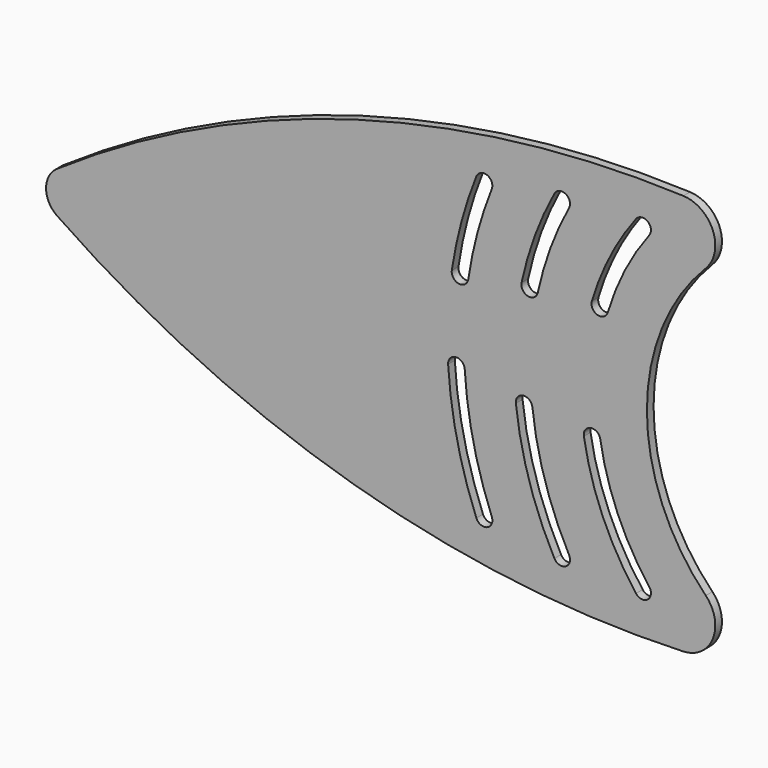
from build123d import *

# Parameters (mm, degrees)
F1_DEPTH = 3.175


# Not quite as in the source:
# - ends of sketch curves that miss each other by under 0.0002 mm in the source are joined


with BuildPart() as f1:
    # F0 (on Front) → F1 (new body)
    with BuildSketch(Plane.XZ):
        with BuildLine():
            ThreePointArc((-123.4070797919, 1.8233010265), (-127.5387969828, -6.0085300089), (-123.4070915827, -13.8403672647))
            ThreePointArc((-123.4070915827, -13.8403672647), (-9.7633198011, -67.3185862363), (114.9359014402, -82.3162835053))
            ThreePointArc((114.9359014402, -82.3162835053), (126.1869378761, -74.3359779231), (123.456379114, -60.815058194))
            ThreePointArc((123.456379114, -60.815058194), (101.0612030172, -6.0085281204), (123.4563821883, 48.798006178))
            ThreePointArc((123.4563821883, 48.798006178), (126.1869343608, 62.3189124907), (114.9359007509, 70.2992174423))
            ThreePointArc((114.9359007509, 70.2992174423), (-9.7633198011, 55.3015372363), (-123.4070797919, 1.8233010265))
        make_face()
        with BuildLine():
            ThreePointArc((77.0821397385, -22.5154604101), (79.7004591586, -18.8888761314), (83.3270330978, -21.5072098724))
            ThreePointArc((83.3270330978, -21.5072098724), (89.9643653266, -44.3549576844), (101.9514625839, -64.9069229437))
            ThreePointArc((101.9514625839, -64.9069229437), (101.3506333254, -69.3393586044), (96.9181875419, -68.7385326678))
            ThreePointArc((96.9181875419, -68.7385326678), (84.1512609661, -46.8495678563), (77.0821397385, -22.5154604101))
        make_face(mode=Mode.SUBTRACT)
        with BuildLine():
            ThreePointArc((25.4272095012, -15.2152278243), (28.3955581041, -11.8691050411), (31.7416808873, -14.837453644))
            ThreePointArc((31.7416808873, -14.837453644), (35.0399400748, -38.2666108744), (42.033430024, -60.8695978255))
            ThreePointArc((42.033430024, -60.8695978255), (40.2700359641, -64.9803081743), (36.1593147519, -63.2169312407))
            ThreePointArc((36.1593147519, -63.2169312407), (28.8665917441, -39.6468400601), (25.4272095012, -15.2152278243))
        make_face(mode=Mode.SUBTRACT)
        with BuildLine():
            ThreePointArc((51.2038323174, -19.8796162989), (54.0078974535, -16.3946587115), (57.4928438898, -19.1987377064))
            ThreePointArc((57.4928438898, -19.1987377064), (62.2856351867, -42.3239729178), (71.4255090517, -64.1003387977))
            ThreePointArc((71.4255090517, -64.1003387977), (70.1400475431, -68.384628042), (65.855751892, -67.099154634))
            ThreePointArc((65.855751892, -67.099154634), (56.24403894, -44.1986400904), (51.2038323174, -19.8796162989))
        make_face(mode=Mode.SUBTRACT)
        with BuildLine():
            ThreePointArc((26.8321292417, 16.6896378099), (30.4920693109, 34.2160200507), (36.1593192267, 51.1998804526))
            ThreePointArc((36.1593192267, 51.1998804526), (40.2700359641, 52.9632591743), (42.0334342681, 48.8525471295))
            ThreePointArc((42.0334342681, 48.8525471295), (36.5987212677, 32.5655461507), (33.0889530651, 15.7582851057))
            ThreePointArc((33.0889530651, 15.7582851057), (29.4948750618, 13.0955480188), (26.8321292417, 16.6896378099))
        make_face(mode=Mode.SUBTRACT)
        with BuildLine():
            ThreePointArc((53.3645508696, 21.2199967221), (58.4187785321, 38.5905299983), (65.8557505543, 55.0821063543))
            ThreePointArc((65.8557505543, 55.0821063543), (70.1400475431, 56.367579042), (71.425520951, 52.0832833909))
            ThreePointArc((71.425520951, 52.0832833909), (64.3536192611, 36.4012543788), (59.5474961242, 19.8834151887))
            ThreePointArc((59.5474961242, 19.8834151887), (55.7877392052, 17.4602445799), (53.3645508696, 21.2199967221))
        make_face(mode=Mode.SUBTRACT)
        with BuildLine():
            ThreePointArc((80.1169824074, 23.7207222996), (87.030580802, 40.9781600378), (96.9181889515, 56.7214825948))
            ThreePointArc((96.9181889515, 56.7214825948), (101.3506333254, 57.3223096044), (101.9514733693, 52.8898657333))
            ThreePointArc((101.9514733693, 52.8898657333), (92.6678111275, 38.108160652), (86.1765020812, 21.9048248522))
            ThreePointArc((86.1765020812, 21.9048248522), (82.2387981181, 19.7830123613), (80.1169824074, 23.7207222996))
        make_face(mode=Mode.SUBTRACT)
    extrude(amount=F1_DEPTH)


solid = f1.part
